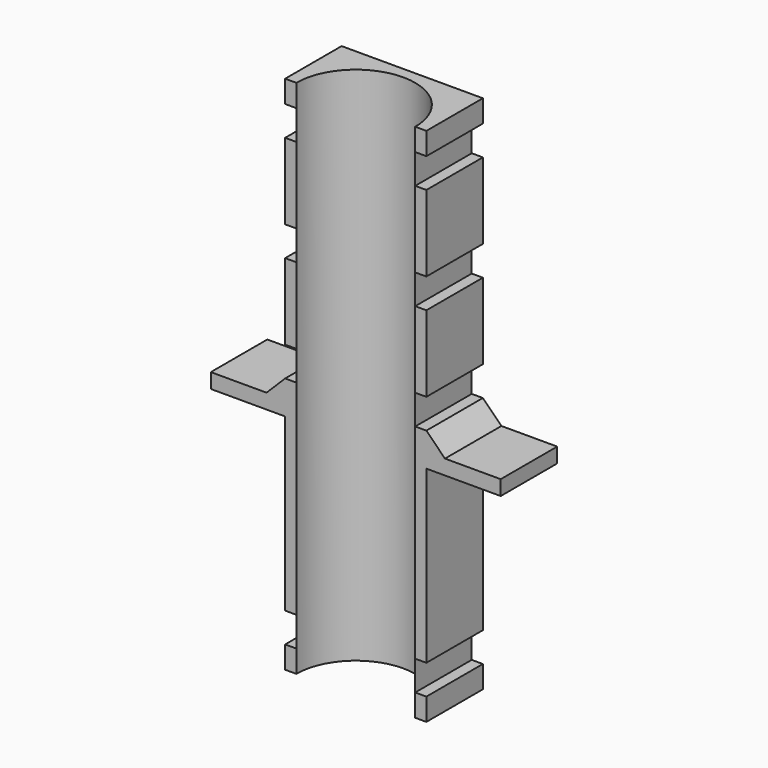
from build123d import *

# Parameters (mm, degrees)
F1_DEPTH = 40
F3_W     = 10
F3_H     = 9.5
F4_DEPTH = 2
F5_DEPTH = 30
F6_W     = 1.5
F6_H     = 4
F7_DEPTH = 9.501
F8_SIZE  = 2.49999


# Not quite as in the source:
# - a fillet or chamfer is up to 0.001 mm smaller than in the source, because OpenCascade refuses the exact size


with BuildPart() as f1:
    # F0 (on Top) → F1 (new body)
    with BuildSketch(Plane.XY):
        with BuildLine():
            Line((-9.5, 0), (-8, 0))
            ThreePointArc((-8, 0), (0, 8), (8, 0))
            Line((8, 0), (9.5, 0))
            Line((9.5, 0), (9.5, 9.5))
            Line((9.5, 9.5), (-9.5, 9.5))
            Line((-9.5, 9.5), (-9.5, 0))
        make_face()
    extrude(amount=-F1_DEPTH)

    # F3 (on offset) → F4 (join)
    with BuildSketch(Plane.XY.offset(-10)):
        with Locations((-14.5, 4.75)):
            Rectangle(F3_W, F3_H)
        with Locations((14.5, 4.75)):
            Rectangle(F3_W, F3_H)
    extrude(amount=F4_DEPTH)

    # F5 (add): a face of the model
    f5_faces = [f1.faces().sort_by_distance(p)[0] for p in [
        (-8.75, 0.2124264579, 0),
    ]]
    extrude(f5_faces, amount=F5_DEPTH)

    # F6 (on face) → F7 (cut, through all)
    with BuildSketch(Plane.XZ):
        with Locations((-8.75, -3.5)):
            Rectangle(F6_W, F6_H)
        with Locations((-8.75, -35)):
            Rectangle(F6_W, F6_H)
        with Locations((8.75, -3.5)):
            Rectangle(F6_W, F6_H)
        with Locations((8.75, -35)):
            Rectangle(F6_W, F6_H)
        with Locations((-8.75, 25)):
            Rectangle(F6_W, F6_H)
        with Locations((8.75, 25)):
            Rectangle(F6_W, F6_H)
        with Locations((-8.75, 10.75)):
            Rectangle(F6_W, F6_H)
        with Locations((8.75, 10.75)):
            Rectangle(F6_W, F6_H)
    extrude(amount=-F7_DEPTH, mode=Mode.SUBTRACT)

    # F8 (size 2.5 in the source; OpenCascade refuses exactly that, so slightly less here)
    f8_edges = [f1.edges().sort_by_distance(p)[0] for p in [
        (-9.5, 4.75, -8),
        (9.5, 4.75, -8),
    ]]
    chamfer(f8_edges, length=F8_SIZE)


solid = f1.part
